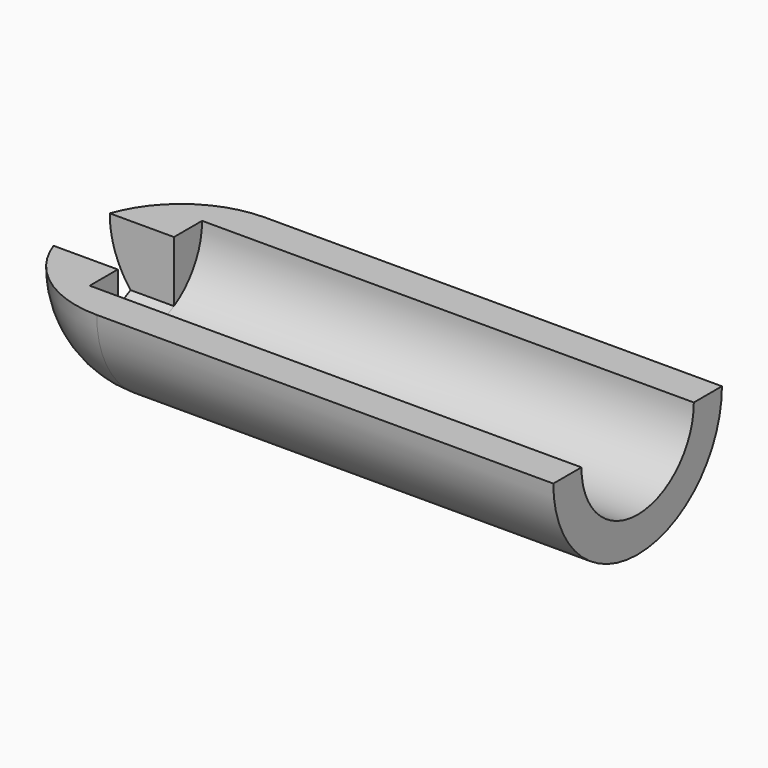
from build123d import *

# Parameters (mm, degrees)
F1_DEPTH = 50.8
F2_R     = 9.52499
F4_DEPTH = 44.45
F6_DEPTH = 6.35


# Not quite as in the source:
# - a fillet or chamfer is up to 0.001 mm smaller than in the source, because OpenCascade refuses the exact size


with BuildPart() as f1:
    # F0 (on Right) → F1 (new body)
    with BuildSketch(Plane.YZ):
        with BuildLine():
            Line((9.525, 0), (-9.525, 0))
            ThreePointArc((-9.525, 0), (0, -9.525), (9.525, 0))
        make_face()
    extrude(amount=F1_DEPTH)

    # F2 (radius 9.525 in the source; OpenCascade refuses exactly that, so slightly less here)
    f2_edges = [f1.edges().sort_by_distance(p)[0] for p in [
        (0, 0, -9.525),
    ]]
    fillet(f2_edges, radius=F2_R)

    # F3 (on face) → F4 (cut)
    with BuildSketch(Plane.YZ.offset(50.8)):
        with BuildLine():
            Line((6.35, 0), (-6.35, 0))
            ThreePointArc((-6.35, 0), (0, -6.35), (6.35, 0))
        make_face()
    extrude(amount=-F4_DEPTH, mode=Mode.SUBTRACT)

    # F5 (on face) → F6 (cut)
    with BuildSketch(Plane.YZ.offset(6.35)):
        with BuildLine():
            Line((3.175, 0), (-3.175, 0))
            Line((-3.175, 0), (-3.175, -5.499261314))
            ThreePointArc((-3.175, -5.499261314), (0, -6.35), (3.175, -5.499261314))
            Line((3.175, -5.499261314), (3.175, 0))
        make_face()
    extrude(amount=-F6_DEPTH, mode=Mode.SUBTRACT)


solid = f1.part
